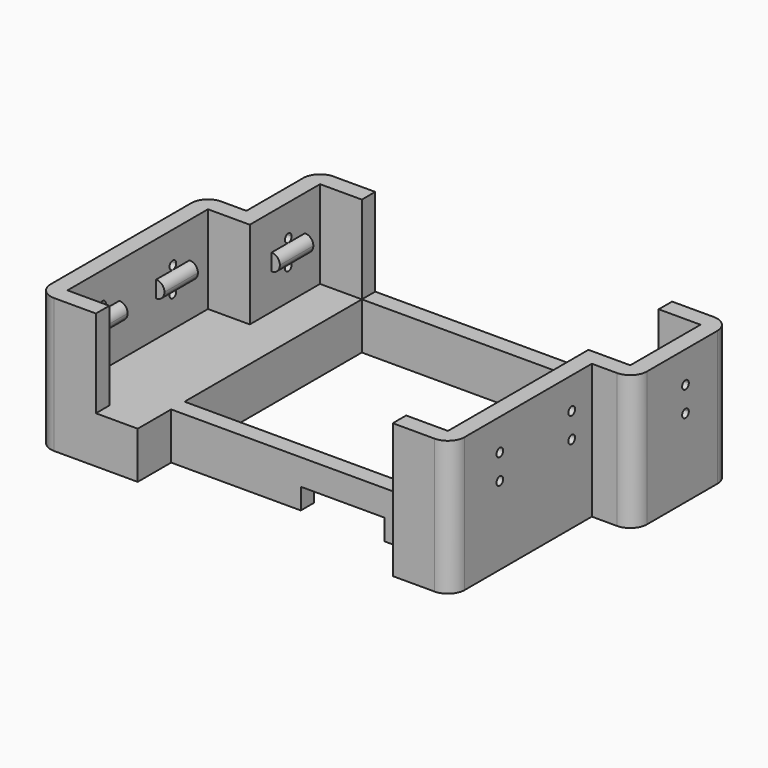
from build123d import *

# Parameters (mm, degrees)
F0_W      = 2
F0_H      = 10.5
F0_H_2    = 2
F0_W_2    = 5
F1_DEPTH  = 16.1
F0_H_3    = 21
F0_W_3    = 30.5
F2_DEPTH  = 5.6
F3_DEPTH  = 5.6
F4_R      = 2
F22_DEPTH = 1
F23_DEPTH = 25
F24_DEPTH = 1
F25_DEPTH = 25
F26_R     = 0.99999
F27_W     = 10
F27_H     = 2.5
F28_DEPTH = 15


# Not quite as in the source:
# - a fillet or chamfer is up to 0.001 mm smaller than in the source, because OpenCascade refuses the exact size


with BuildPart() as f1:
    # F0 (on Top) → F1 (new body)
    with BuildSketch(Plane.XY):
        with Locations((53.5, 28.25)):
            Rectangle(F0_W, F0_H)
        with Locations((53.5, 34.5)):
            Rectangle(F0_W, F0_H_2)
        Polygon((52.5, 23), (49.5, 23), (49.5, 21), (54.5, 21), (54.5, 23), align=None)
        Polygon((47.5, 23), (47.5, 2), (49.5, 2), (49.5, 21), (49.5, 23), align=None)
        with Locations((48.5, 1)):
            Rectangle(F0_W, F0_H_2)
        with Locations((45, 1)):
            Rectangle(F0_W_2, F0_H_2)
        with Locations((50, 34.5)):
            Rectangle(F0_W_2, F0_H_2)
    extrude(amount=F1_DEPTH)



with BuildPart() as f1b:
    # F0 (on Top) → F1, piece 2 (new body)
    with BuildSketch(Plane.XY):
        with Locations((6, 34.5)):
            Rectangle(F0_W, F0_H_2)
        Polygon((5, 25), (5, 23), (7, 23), (7, 33.5), (5, 33.5), align=None)
        Polygon((0, 25), (0, 23), (2, 23), (5, 23), (5, 25), align=None)
        with Locations((1, 12.5)):
            Rectangle(F0_W, F0_H_3)
        with Locations((1, 1)):
            Rectangle(F0_W, F0_H_2)
        with Locations((4.5, 1)):
            Rectangle(F0_W_2, F0_H_2)
        with Locations((9.5, 34.5)):
            Rectangle(F0_W_2, F0_H_2)
    extrude(amount=F1_DEPTH)


with BuildPart() as f1_1:
    add(f1.part)

    add(f1b.part)  # F2 merges F1b
    # F0 (on Top) → F2 (join)
    with BuildSketch(Plane.XY):
        with Locations((27.25, 34.5)):
            Rectangle(F0_W_3, F0_H_2)
        with Locations((45, 34.5)):
            Rectangle(F0_W_2, F0_H_2)
        with Locations((9.5, 1)):
            Rectangle(F0_W_2, F0_H_2)
        Polygon((2, 23), (2, 2), (7, 2), (7, 23), (5, 23), align=None)
        Polygon((7, 23), (7, 2), (12, 2), (12, 5), (12, 7), (12, 23), align=None)
        with Locations((9.5, 28.25)):
            Rectangle(F0_W_2, F0_H)
        Polygon((42.5, 33.5), (42.5, 23), (47.5, 23), (49.5, 23), (52.5, 23), (52.5, 33.5), (47.5, 33.5), align=None)
        Polygon((42.5, 5), (42.5, 2), (47.5, 2), (47.5, 23), (42.5, 23), (42.5, 7), align=None)
    extrude(amount=F2_DEPTH)

    # F0 (on Top) → F3 (join)
    with BuildSketch(Plane.XY):
        with Locations((27.25, 6)):
            Rectangle(F0_W_3, F0_H_2)
    extrude(amount=F3_DEPTH)

    # F4
    f4_edges = [f1_1.edges().sort_by_distance(p)[0] for p in [
        (0, 0, 8.05),
        (0, 25, 8.05),
        (5, 35.5, 8.05),
        (54.5, 35.5, 8.05),
        (54.5, 21, 8.05),
        (49.5, 0, 8.05),
    ]]
    fillet(f4_edges, radius=F4_R)

    # F18 (on 3pt) + F19 (on 3pt) → F22 (join)
    with BuildSketch(Plane.YZ.offset(2)):
        Polygon((4.75, 11.85), (4.75, 9.85), (7.25, 9.85), (9.75, 9.85), (9.75, 11.85), (7.25, 11.85), align=None)
        Polygon((15.25, 11.85), (15.25, 9.85), (17.75, 9.85), (20.25, 9.85), (20.25, 11.85), (17.75, 11.85), align=None)
    with BuildSketch(Plane.YZ.offset(7)):
        Polygon((26.25, 11.85), (26.25, 9.85), (28.75, 9.85), (31.25, 9.85), (31.25, 11.85), (28.75, 11.85), align=None)
    extrude(amount=F22_DEPTH)

    # F18 (on 3pt) + F19 (on 3pt) → F23 (cut)
    with BuildSketch(Plane.YZ.offset(2)):
        with BuildLine():
            ThreePointArc((18.25, 12.35), (17.3964466094, 12.7035533906), (17.75, 11.85))
            ThreePointArc((17.75, 11.85), (18.1035533906, 11.9964466094), (18.25, 12.35))
        make_face()
        with BuildLine():
            ThreePointArc((18.25, 9.35), (18.1035533906, 9.7035533906), (17.75, 9.85))
            ThreePointArc((17.75, 9.85), (17.3964466094, 8.9964466094), (18.25, 9.35))
        make_face()
        with BuildLine():
            ThreePointArc((7.75, 9.35), (7.6035533906, 9.7035533906), (7.25, 9.85))
            ThreePointArc((7.25, 9.85), (6.8964466094, 8.9964466094), (7.75, 9.35))
        make_face()
        with BuildLine():
            ThreePointArc((7.75, 12.35), (6.8964466094, 12.7035533906), (7.25, 11.85))
            ThreePointArc((7.25, 11.85), (7.6035533906, 11.9964466094), (7.75, 12.35))
        make_face()
    with BuildSketch(Plane.YZ.offset(7)):
        with BuildLine():
            ThreePointArc((29.25, 12.35), (28.3964466094, 12.7035533906), (28.75, 11.85))
            ThreePointArc((28.75, 11.85), (29.1035533906, 11.9964466094), (29.25, 12.35))
        make_face()
        with BuildLine():
            ThreePointArc((29.25, 9.35), (29.1035533906, 9.7035533906), (28.75, 9.85))
            ThreePointArc((28.75, 9.85), (28.3964466094, 8.9964466094), (29.25, 9.35))
        make_face()
    extrude(amount=-F23_DEPTH, mode=Mode.SUBTRACT)

    # F20 (on 3pt) + F21 (on 3pt) → F24 (join)
    with BuildSketch(Plane(origin=(47.5, 0, 0), x_dir=(0, -1, 0), z_dir=(-1, 0, 0))):
        Polygon((-20.5, 11.85), (-20.5, 9.85), (-18, 9.85), (-15.5, 9.85), (-15.5, 11.85), (-18, 11.85), align=None)
        Polygon((-9.75, 11.85), (-9.75, 9.85), (-7.25, 9.85), (-4.75, 9.85), (-4.75, 11.85), (-7.25, 11.85), align=None)
    with BuildSketch(Plane.YZ.offset(52.5)):
        Polygon((26.25, 11.85), (26.25, 9.85), (28.75, 9.85), (31.25, 9.85), (31.25, 11.85), (28.75, 11.85), align=None)
    extrude(amount=F24_DEPTH, dir=(-1, 0, 0))

    # F21 (on 3pt) + F20 (on 3pt) → F25 (cut)
    with BuildSketch(Plane.YZ.offset(52.5)):
        with BuildLine():
            ThreePointArc((29.25, 12.35), (28.3964466094, 12.7035533906), (28.75, 11.85))
            ThreePointArc((28.75, 11.85), (29.1035533906, 11.9964466094), (29.25, 12.35))
        make_face()
        with BuildLine():
            ThreePointArc((29.25, 9.35), (29.1035533906, 9.7035533906), (28.75, 9.85))
            ThreePointArc((28.75, 9.85), (28.3964466094, 8.9964466094), (29.25, 9.35))
        make_face()
    with BuildSketch(Plane(origin=(47.5, 0, 0), x_dir=(0, -1, 0), z_dir=(-1, 0, 0))):
        with BuildLine():
            ThreePointArc((-17.5, 12.35), (-18.3535533906, 12.7035533906), (-18, 11.85))
            ThreePointArc((-18, 11.85), (-17.6464466094, 11.9964466094), (-17.5, 12.35))
        make_face()
        with BuildLine():
            ThreePointArc((-17.5, 9.35), (-17.6464466094, 9.7035533906), (-18, 9.85))
            ThreePointArc((-18, 9.85), (-18.3535533906, 8.9964466094), (-17.5, 9.35))
        make_face()
        with BuildLine():
            ThreePointArc((-6.75, 12.35), (-7.6035533906, 12.7035533906), (-7.25, 11.85))
            ThreePointArc((-7.25, 11.85), (-6.8964466094, 11.9964466094), (-6.75, 12.35))
        make_face()
        with BuildLine():
            ThreePointArc((-6.75, 9.35), (-6.8964466094, 9.7035533906), (-7.25, 9.85))
            ThreePointArc((-7.25, 9.85), (-7.6035533906, 8.9964466094), (-6.75, 9.35))
        make_face()
    extrude(amount=F25_DEPTH, dir=(1, 0, 0), mode=Mode.SUBTRACT)

    # F26 (radius 1 in the source; OpenCascade refuses exactly that, so slightly less here)
    f26_edges = [f1_1.edges().sort_by_distance(p)[0] for p in [
        (3, 7.25, 11.85),
        (3, 7.25, 9.85),
        (3, 17.75, 11.85),
        (3, 17.75, 9.85),
        (8, 28.75, 11.85),
        (8, 28.75, 9.85),
        (46.5, 18, 9.85),
        (46.5, 7.25, 9.85),
        (46.5, 7.25, 11.85),
        (46.5, 18, 11.85),
        (51.5, 28.75, 11.85),
        (51.5, 28.75, 9.85),
    ]]
    fillet(f26_edges, radius=F26_R)

    # F27 (on face) → F28 (cut)
    with BuildSketch(Plane.XZ.offset(-5)):
        with Locations((32.5, 1.25)):
            Rectangle(F27_W, F27_H)
    extrude(amount=-F28_DEPTH, mode=Mode.SUBTRACT)


solid = f1_1.part
